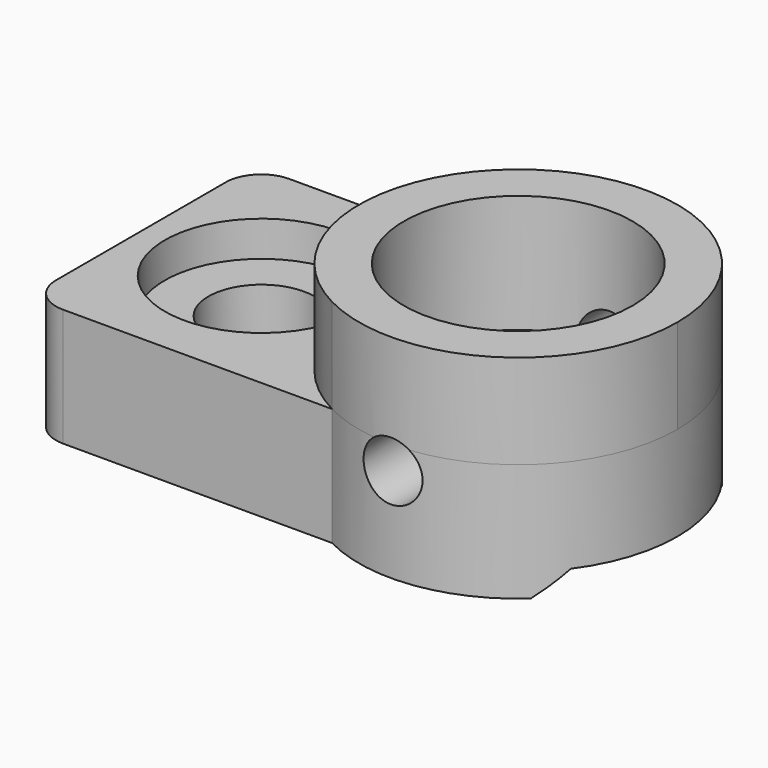
from build123d import *

# Parameters (mm, degrees)
F1_DEPTH  = 5
F3_DEPTH  = 22.751
F4_R      = 2.25
F5_DEPTH  = 25
F6_R      = 4.1
F6_R_2    = 2.25
F7_DEPTH  = 1.5
F9_DEPTH  = 4
F10_R     = 1.5
F11_R     = 4.85
F12_DEPTH = 5
F13_R     = 1.25
F14_DEPTH = 12.5


# Not quite as in the source:
# - a feature names something its author has since deleted; it is built from what else it names


with BuildPart() as f1:
    # F0 (on Top) → F1 (new body)
    with BuildSketch(Plane.XY):
        with BuildLine():
            Line((-10.5, -6), (2.4076707808, -6))
            ThreePointArc((2.4076707808, -6), (12.25, 0), (2.4076707808, 6))
            Line((2.4076707808, 6), (-10.5, 6))
            Line((-10.5, 6), (-10.5, -6))
        make_face()
    extrude(amount=F1_DEPTH)

    # F2 (on face) → F3 (cut, through all)
    with BuildSketch(Plane(origin=(-10.5, 0, 0), x_dir=(0, -1, 0), z_dir=(-1, 0, 0))):
        Polygon((5, 0), (4, 1), (-4, 1), (-5, 0), align=None)
    extrude(amount=-F3_DEPTH, mode=Mode.SUBTRACT)

    # F4 (on face) → F5 (cut)
    with BuildSketch(Plane.XY.offset(5)):
        with Locations((-5.3849667311, 0)):
            Circle(F4_R)
    extrude(amount=-F5_DEPTH, mode=Mode.SUBTRACT)

    # F6 (on face) → F7 (cut)
    with BuildSketch(Plane.XY.offset(5)):
        with Locations((-5.3849667311, 0)):
            Circle(F6_R)
        with Locations((-5.3849667311, 0)):
            Circle(F6_R_2, mode=Mode.SUBTRACT)
    extrude(amount=-F7_DEPTH, mode=Mode.SUBTRACT)

    # F8 (on face) → F9 (join)
    with BuildSketch(Plane.XY.offset(5)):
        with BuildLine():
            ThreePointArc((2.4076707808, -6), (9.0134938288, -5.7634938288), (12.25, 0))
            ThreePointArc((12.25, 0), (9.0134938288, 5.7634938288), (2.4076707808, 6))
            ThreePointArc((2.4076707808, 6), (-1.25, 0), (2.4076707808, -6))
        make_face()
    extrude(amount=F9_DEPTH)

    # F10
    f10_edges = [f1.edges().sort_by_distance(p)[0] for p in [
        (-10.5, -6, 2.5),
        (-10.5, 6, 2.5),
    ]]
    fillet(f10_edges, radius=F10_R)

    # F11 (on face) → F12 (cut)
    with BuildSketch(Plane.XY.offset(9)):
        with Locations((5.5, 0)):
            Circle(F11_R)
    extrude(amount=-F12_DEPTH, mode=Mode.SUBTRACT)

    # F13 (on Front) → F14 (cut, symmetric)
    with BuildSketch(Plane.XZ):
        with Locations((5.5, 4)):
            Circle(F13_R)
    extrude(amount=F14_DEPTH, both=True, mode=Mode.SUBTRACT)


solid = f1.part
